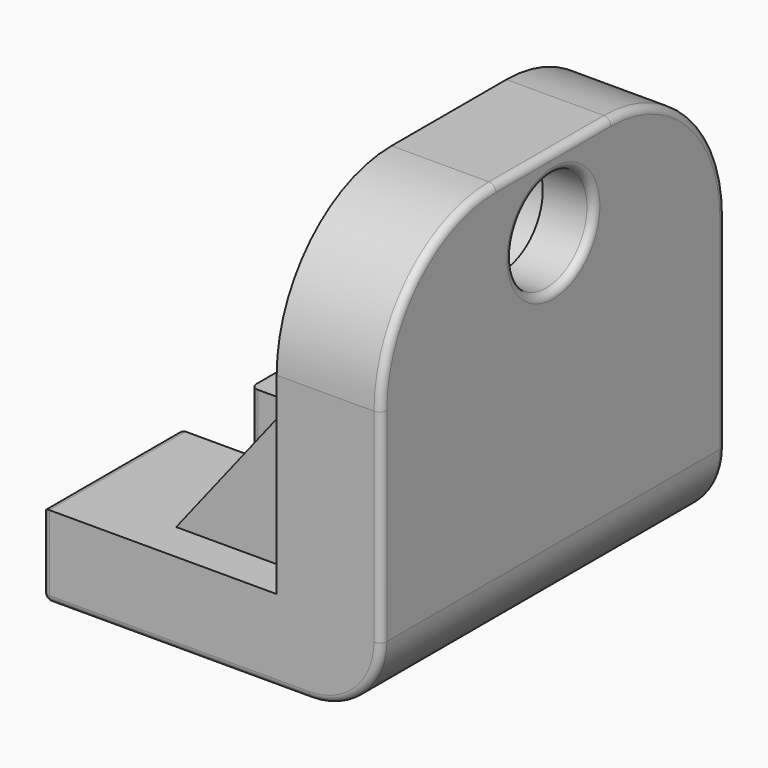
from build123d import *

# Parameters (mm, degrees)
F1_DEPTH  = 38.1
F2_R      = 9.0076691871
F3_DEPTH  = 18.4852466609
F4_R      = 11.43
F4_R_2    = 9.0076691871
F6_DEPTH  = 9.398
F7_DEPTH  = 25.4
F10_DEPTH = 5.715
F12_R     = 25.4
F13_R     = 12.7
F14_R     = 1.27


# Not quite as in the source:
# - a pattern or mirror of a feature is missing from the dataset's text; its kind, count and spacing are read off the source's solid


with BuildPart() as f1:
    # F0 (on Front) → F1 (new body, symmetric)
    with BuildSketch(Plane.XZ):
        Polygon((0, 0), (0, 74.0791857243), (-18.4852466609, 74.0791857243), (-18.4852466609, 14.5855043083), (-59.9480941892, 14.5855043083), (-59.9480941892, 0), align=None)
    extrude(amount=F1_DEPTH, both=True)

    # F2 (on face) → F3 (cut, through all)
    with BuildSketch(Plane(origin=(-18.4852466609, 0, 0), x_dir=(0, -1, 0), z_dir=(-1, 0, 0))):
        with Locations((0, 61.3791857243)):
            Circle(F2_R)
    extrude(amount=-F3_DEPTH, mode=Mode.SUBTRACT)

    # F4 (on face) → F6 (cut)
    with BuildSketch(Plane(origin=(-18.4852466609, 0, 0), x_dir=(0, -1, 0), z_dir=(-1, 0, 0))):
        with Locations((0, 61.3791857243)):
            Circle(F4_R)
        with Locations((0, 61.3791857243)):
            Circle(F4_R_2, mode=Mode.SUBTRACT)
    extrude(amount=-F6_DEPTH, mode=Mode.SUBTRACT)

    # F5 (on face) → F7 (cut)
    with BuildSketch(Plane.XY.offset(14.5855043083)):
        with BuildLine():
            ThreePointArc((-47.9387399794, -8.003022201), (-55.2808618291, 0), (-47.9387399794, 8.003022201))
            Line((-47.9387399794, 8.003022201), (-59.9480941892, 8.003022201))
            Line((-59.9480941892, 8.003022201), (-59.9480941892, -8.003022201))
            Line((-59.9480941892, -8.003022201), (-47.9387399794, -8.003022201))
        make_face()
        with BuildLine():
            ThreePointArc((-47.9387399794, -8.003022201), (-41.8177369816, -5.9191702591), (-39.2153265492, 0))
            ThreePointArc((-39.2153265492, 0), (-41.8177369816, 5.9191702591), (-47.9387399794, 8.003022201))
            ThreePointArc((-47.9387399794, 8.003022201), (-55.2808618291, 0), (-47.9387399794, -8.003022201))
        make_face()
    extrude(amount=-F7_DEPTH, mode=Mode.SUBTRACT)

    # F9 (on offset) → F10 (join, symmetric)
    with BuildSketch(Plane.XZ.offset(25.4)):
        Polygon((-41.8496876955, 14.5855043083), (-18.4852466609, 14.5855043083), (-18.4852466609, 44.3323450163), align=None)
    f10 = extrude(amount=F10_DEPTH, both=True)

    # F10_copies: F10 across plane
    add(f10.mirror(Plane.ZX))

    # F12
    f12_edges = [f1.edges().sort_by_distance(p)[0] for p in [
        (-9.242623, 38.1, 74.079186),
        (-9.242623, -38.1, 74.079186),
    ]]
    fillet(f12_edges, radius=F12_R)

    # F13
    f13_edges = [f1.edges().sort_by_distance(p)[0] for p in [
        (0, 0, 0),
    ]]
    fillet(f13_edges, radius=F13_R)

    # F14
    f14_edges = [f1.edges().sort_by_distance(p)[0] for p in [
        (0, 38.1, 30.689593),
        (0, 0, 12.7),
        (0, 30.660512, 66.639698),
        (0, -38.1, 30.689593),
        (0, 0, 74.079186),
        (0, -30.660512, 66.639698),
        (0, 9.007669, 61.379186),
        (-59.948094, 23.051511, 0),
        (-3.719744, 38.1, 3.719744),
        (-36.324047, 38.1, 0),
        (-3.719744, -38.1, 3.719744),
        (-36.324047, -38.1, 0),
        (-59.948094, -38.1, 7.292752),
        (-59.948094, -23.051511, 0),
        (-59.948094, 8.003022, 7.292752),
        (-59.948094, -23.051511, 14.585504),
        (-59.948094, -8.003022, 7.292752),
    ]]
    fillet(f14_edges, radius=F14_R)


solid = f1.part
